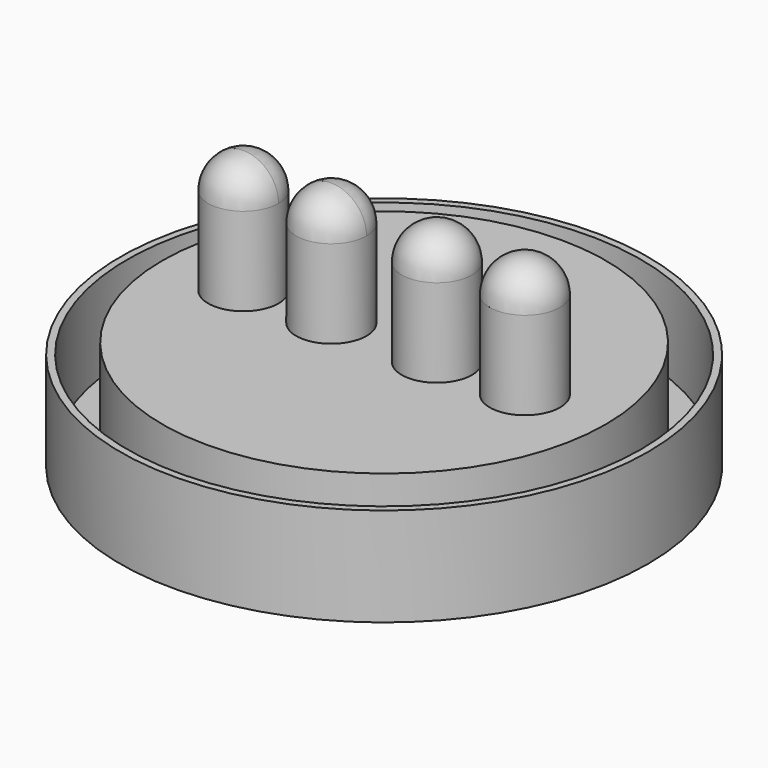
from build123d import *
from build123d import SkipClean  # not in build123d's __all__

# Parameters (mm, degrees)
F0_R     = 75
F0_R_2   = 73
F0_R_3   = 63
F0_R_4   = 61
F1_DEPTH = 3
F2_R     = 75
F2_R_2   = 73
F2_R_3   = 63
F2_R_4   = 61
F3_DEPTH = 25
F4_DEPTH = 3
F5_R     = 63
F5_R_2   = 61
F6_DEPTH = 3
F7_R     = 10
F8_DEPTH = 25


with BuildPart() as f1:
    # F0 (on Top) → F1 (new body)
    with BuildSketch(Plane.XY):
        Circle(F0_R)
        Circle(F0_R_2, mode=Mode.SUBTRACT)
        Circle(F0_R_2)
        Circle(F0_R_3, mode=Mode.SUBTRACT)
        Circle(F0_R_3)
        Circle(F0_R_4, mode=Mode.SUBTRACT)
    extrude(amount=F1_DEPTH)

    # F2 (on face) → F3 (join)
    with BuildSketch(Plane.XY.offset(3)):
        Circle(F2_R)
        Circle(F2_R_2, mode=Mode.SUBTRACT)
        Circle(F2_R_3)
        Circle(F2_R_4, mode=Mode.SUBTRACT)
    extrude(amount=F3_DEPTH)

    # F0 (on Top) → F4 (join)
    with BuildSketch(Plane.XY):
        Circle(F0_R_4)
    extrude(amount=F4_DEPTH)

    # F5 (on face) → F6 (join)
    with BuildSketch(Plane.XY.offset(28)):
        Circle(F5_R)
        Circle(F5_R_2, mode=Mode.SUBTRACT)
        Circle(F5_R_2)
    extrude(amount=F6_DEPTH)


with BuildPart() as f8:
    # F7 (on face) → F8 (new body)
    with BuildSketch(Plane.XY.offset(31)):
        with Locations((-40, 0)):
            Circle(F7_R)
    extrude(amount=F8_DEPTH)

    # F9 (on Front) → F10 (revolve)
    with BuildSketch(Plane.XZ):
        with BuildLine():
            ThreePointArc((-30, 56), (-40, 66), (-50, 56))
            Line((-50, 56), (-30, 56))
        make_face()
    with SkipClean():  # cleaning this boolean's faces spoils the solid; the shape is the same uncleaned
        revolve(axis=Axis((-40, 0, 56), (1, 0, 0)))


with BuildPart() as f8b:
    # F7 (on face) → F8, piece 2 (new body)
    with BuildSketch(Plane.XY.offset(31)):
        with Locations((-15, 0)):
            Circle(F7_R)
    extrude(amount=F8_DEPTH)

    # F9 (on Front) → F11 (revolve)
    with BuildSketch(Plane.XZ):
        with BuildLine():
            ThreePointArc((-5, 56), (-15, 66), (-25, 56))
            Line((-25, 56), (-5, 56))
        make_face()
    with SkipClean():  # cleaning this boolean's faces spoils the solid; the shape is the same uncleaned
        revolve(axis=Axis((-15, 0, 56), (1, 0, 0)))


with BuildPart() as f8c:
    # F7 (on face) → F8, piece 3 (new body)
    with BuildSketch(Plane.XY.offset(31)):
        with Locations((15, 0)):
            Circle(F7_R)
    extrude(amount=F8_DEPTH)

    # F9 (on Front) → F12 (revolve)
    with BuildSketch(Plane.XZ):
        with BuildLine():
            Line((5, 56), (25, 56))
            ThreePointArc((25, 56), (15, 66), (5, 56))
        make_face()
    revolve(axis=Axis((15, 0, 56), (-1, 0, 0)))


with BuildPart() as f8d:
    # F7 (on face) → F8, piece 4 (new body)
    with BuildSketch(Plane.XY.offset(31)):
        with Locations((40, 0)):
            Circle(F7_R)
    extrude(amount=F8_DEPTH)

    # F9 (on Front) → F13 (revolve)
    with BuildSketch(Plane.XZ):
        with BuildLine():
            Line((30, 56), (50, 56))
            ThreePointArc((50, 56), (40, 66), (30, 56))
        make_face()
    revolve(axis=Axis((40, 0, 56), (-1, 0, 0)))


solid = Compound([f1.part, f8.part, f8b.part, f8c.part, f8d.part])
